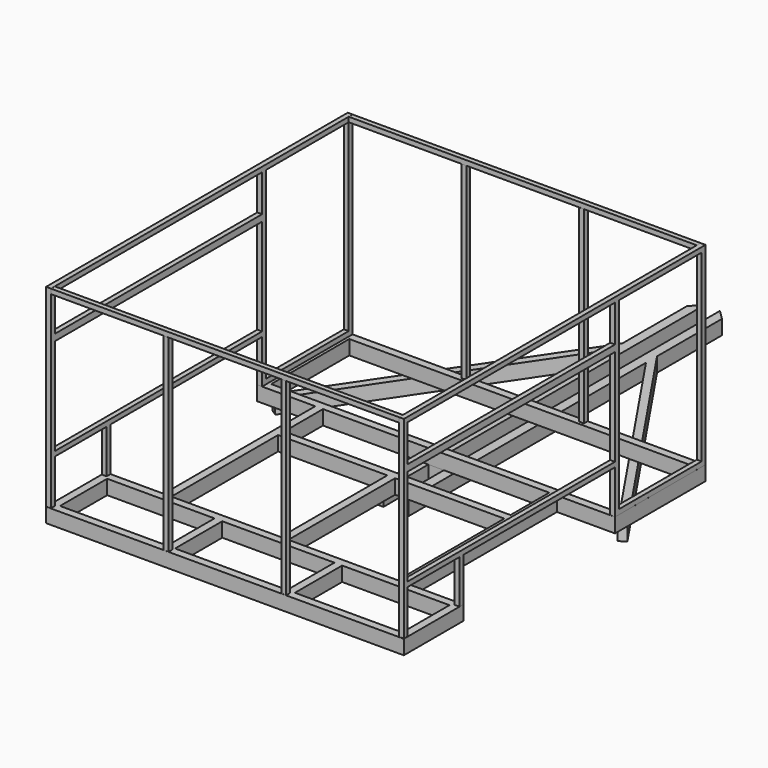
from build123d import *

# Parameters (mm, degrees)
F0_W      = 50
F0_H      = 40
F0_W_2    = 80
F0_W_3    = 495
F0_W_4    = 40
F0_H_2    = 689.5836830139
F0_H_3    = 305
F1_DEPTH  = 75
F0_H_4    = 250.4163169861
F0_H_5    = 505
F2_DEPTH  = 75
F3_W      = 535
F3_H      = 951
F3_W_2    = 25
F3_H_2    = 225.9821975827
F3_W_3    = 1340
F3_H_3    = 33.8248362541
F4_DEPTH  = 25
F7_W      = 1340
F7_H      = 33.8248362541
F7_W_2    = 535
F7_H_2    = 951
F7_W_3    = 25
F7_H_3    = 225.9821975827
F8_DEPTH  = 25
F9_W      = 25
F9_H      = 975.6403267384
F10_DEPTH = 25
F12_DEPTH = 25
F11_W     = 25
F11_H     = 975.6403267384


# Not quite as in the source:
# - a feature names something its author has since deleted; it is built from what else it names


with BuildPart() as f1:
    # F0 (on Top) → F1 (new body)
    with BuildSketch(Plane.XY):
        Polygon((341.9006320566, 0), (0, 0), (0, -585), (300, -585), (340, -585), (835, -585), (835, -545), (40, -545), (40, -518.7423229218), (6.8463404132, -496.362982985), (40, -447.2478103703), (40, -40), (314.8998843676, -40), align=None)
        Polygon((390.1607644204, 0), (341.9006320566, 0), (314.8998843676, -40), (363.1600167314, -40), align=None)
        Polygon((835, 0), (390.1607644204, 0), (363.1600167314, -40), (835, -40), align=None)
        Polygon((340, -585), (300, -585), (300, -1565), (340, -1565), (340, -875.4163169861), (340, -835.4163169861), align=None)
        with Locations((860, -20)):
            Rectangle(F0_W, F0_H)
        Polygon((40, -518.7423229218), (40, -447.2478103703), (6.8463404132, -496.362982985), align=None)
        Polygon((340, -1565), (300, -1565), (0, -1565), (0, -1950), (1850, -1950), (1850, -1565), (1550, -1565), (1510, -1565), (945, -1565), (905, -1565), align=None)
        Polygon((1255, -1605), (1810, -1605), (1810, -1910), (1255, -1910), (1215, -1910), (635, -1910), (595, -1910), (40, -1910), (40, -1605), (595, -1605), (635, -1605), (1215, -1605), align=None, mode=Mode.SUBTRACT)
        with Locations((925, -20)):
            Rectangle(F0_W_2, F0_H)
        with Locations((860, -565)):
            Rectangle(F0_W, F0_H)
        with Locations((587.5, -855.4163169861)):
            Rectangle(F0_W_3, F0_H)
        with Locations((990, -20)):
            Rectangle(F0_W, F0_H)
        with Locations((925, -565)):
            Rectangle(F0_W_2, F0_H)
        with Locations((860, -855.4163169861)):
            Rectangle(F0_W, F0_H)
        with Locations((925, -1220.208158493)):
            Rectangle(F0_W_4, F0_H_2)
        Polygon((1459.8392355796, 0), (1015, 0), (1015, -40), (1486.8399832686, -40), align=None)
        with Locations((990, -565)):
            Rectangle(F0_W, F0_H)
        Polygon((965, -835.4163169861), (885, -835.4163169861), (885, -875.4163169861), (905, -875.4163169861), (945, -875.4163169861), (965, -875.4163169861), align=None)
        Polygon((1508.0993679434, 0), (1459.8392355796, 0), (1486.8399832686, -40), (1535.1001156324, -40), align=None)
        Polygon((1015, -545), (1015, -585), (1510, -585), (1550, -585), (1850, -585), (1850, 0), (1508.0993679434, 0), (1535.1001156324, -40), (1810, -40), (1810, -447.2478103703), (1843.1536595868, -496.362982985), (1810, -518.7423229218), (1810, -545), align=None)
        with Locations((990, -855.4163169861)):
            Rectangle(F0_W, F0_H)
        Polygon((1510, -875.4163169861), (1510, -1565), (1550, -1565), (1550, -585), (1510, -585), (1510, -835.4163169861), align=None)
        with Locations((1262.5, -855.4163169861)):
            Rectangle(F0_W_3, F0_H)
        Polygon((1810, -447.2478103703), (1810, -518.7423229218), (1843.1536595868, -496.362982985), align=None)
        with Locations((1235, -1757.5)):
            Rectangle(F0_W_4, F0_H_3)
        with Locations((615, -1757.5)):
            Rectangle(F0_W_4, F0_H_3)
    extrude(amount=F1_DEPTH)


with BuildPart() as f2:
    # F0 (on Top) → F2 (new body)
    with BuildSketch(Plane.XY):
        with Locations((990, -710.208158493)):
            Rectangle(F0_W, F0_H_4)
        Polygon((835, 730.4973530704), (341.9006320566, 0), (390.1607644204, 0), (835, 659.0028405189), align=None)
        Polygon((363.1600167314, -40), (314.8998843676, -40), (40, -447.2478103703), (40, -518.7423229218), align=None)
        Polygon((390.1607644204, 0), (341.9006320566, 0), (314.8998843676, -40), (363.1600167314, -40), align=None)
        with Locations((990, -292.5)):
            Rectangle(F0_W, F0_H_5)
        Polygon((1535.1001156324, -40), (1486.8399832686, -40), (1810, -518.7423229218), (1810, -447.2478103703), align=None)
        Polygon((1015, 659.0028405189), (1459.8392355796, 0), (1508.0993679434, 0), (1015, 730.4973530704), align=None)
        Polygon((1508.0993679434, 0), (1459.8392355796, 0), (1486.8399832686, -40), (1535.1001156324, -40), align=None)
        with Locations((990, -20)):
            Rectangle(F0_W, F0_H)
        with Locations((860, -20)):
            Rectangle(F0_W, F0_H)
        with Locations((860, -565)):
            Rectangle(F0_W, F0_H)
        with Locations((925, -565)):
            Rectangle(F0_W_2, F0_H)
        with Locations((990, -565)):
            Rectangle(F0_W, F0_H)
        with Locations((860, -855.4163169861)):
            Rectangle(F0_W, F0_H)
        with Locations((990, -855.4163169861)):
            Rectangle(F0_W, F0_H)
        Polygon((40, -518.7423229218), (40, -447.2478103703), (6.8463404132, -496.362982985), align=None)
        Polygon((1810, -447.2478103703), (1810, -518.7423229218), (1843.1536595868, -496.362982985), align=None)
        with Locations((860, -292.5)):
            Rectangle(F0_W, F0_H_5)
        with Locations((860, -710.208158493)):
            Rectangle(F0_W, F0_H_4)
        Polygon((835, 1150), (835, 730.4973530704), (835, 659.0028405189), (835, 0), (885, 0), (885, 1200), align=None)
        Polygon((965, 1200), (965, 0), (1015, 0), (1015, 659.0028405189), (1015, 730.4973530704), (1015, 1150), align=None)
    extrude(amount=-F2_DEPTH)


with BuildPart() as f4:
    # F3 (on Right) → F4 (new body)
    with BuildSketch(Plane.YZ):
        Polygon((0, 75.0093311071), (0, 1076), (-1950, 1076), (-1950, 76), (-1925, 76), (-1925, 301), (-1925, 326), (-1925, 826), (-1925, 859.8248362541), (-1925, 1051), (-585, 1051), (-585, 859.8248362541), (-585, 826), (-585, 326), (-585, 301), (-585, 75.0093311071), align=None)
        with Locations((-292.5, 575.5)):
            Rectangle(F3_W, F3_H, mode=Mode.SUBTRACT)
        Polygon((-1565, 301), (-585, 301), (-585, 326), (-1925, 326), (-1925, 301), (-1590, 301), align=None)
        with Locations((-1577.5, 188.0089012086)):
            Rectangle(F3_W_2, F3_H_2)
        with Locations((-1255, 842.9124181271)):
            Rectangle(F3_W_3, F3_H_3)
    extrude(amount=F4_DEPTH)


with BuildPart() as f8:
    # F7 (on offset) → F8 (new body)
    with BuildSketch(Plane.YZ.offset(1850)):
        with Locations((-1254.9842073394, 842.9438270557)):
            Rectangle(F7_W, F7_H)
        Polygon((0.0157926606, 75.0407400358), (0.0157926606, 1076.0314089287), (-1949.9842073394, 1076.0314089287), (-1949.9842073394, 76.0314089287), (-1924.9842073394, 76.0314089287), (-1924.9842073394, 301.0314089287), (-1924.9842073394, 326.0314089287), (-1924.9842073394, 826.0314089287), (-1924.9842073394, 859.8562451828), (-1924.9842073394, 1051.0314089287), (-584.9842073394, 1051.0314089287), (-584.9842073394, 859.8562451828), (-584.9842073394, 826.0314089287), (-584.9842073394, 326.0314089287), (-584.9842073394, 301.0314089287), (-584.9842073394, 75.0407400358), align=None)
        with Locations((-292.4842073394, 575.5314089287)):
            Rectangle(F7_W_2, F7_H_2, mode=Mode.SUBTRACT)
        Polygon((-1564.9842073394, 301.0314089287), (-584.9842073394, 301.0314089287), (-584.9842073394, 326.0314089287), (-1924.9842073394, 326.0314089287), (-1924.9842073394, 301.0314089287), (-1589.9842073394, 301.0314089287), align=None)
        with Locations((-1577.4842073394, 188.0403101373)):
            Rectangle(F7_W_3, F7_H_3)
    extrude(amount=-F8_DEPTH)


with BuildPart() as f10:
    # F9 (on Front) → F10 (new body)
    with BuildSketch(Plane.XZ):
        with Locations((1229.0860442189, 563.0803654591)):
            Rectangle(F9_W, F9_H)
    extrude(amount=F10_DEPTH)


with BuildPart() as f10b:
    # F9 (on Front) → F10, piece 2 (new body)
    with BuildSketch(Plane.XZ):
        with Locations((620.7860442189, 563.0803654591)):
            Rectangle(F9_W, F9_H)
    extrude(amount=F10_DEPTH)


with BuildPart() as f10c:
    # F9 (on Front) → F10, piece 3 (new body)
    with BuildSketch(Plane.XZ):
        Polygon((25.0013015178, 1075.9552220504), (24.9906565008, 1050.9557227294), (1824.9834692982, 1050.9557227294), (1824.9834692982, 1076.006124417), align=None)
    extrude(amount=F10_DEPTH)


with BuildPart() as f12:
    # F11 (on offset) → F12 (new body)
    with BuildSketch(Plane.XZ.offset(1950)):
        Polygon((25.0165007023, 1075.9785572688), (25.0058556852, 1050.9790579478), (1824.9986684827, 1050.9790579478), (1824.9986684827, 1076.0294596354), align=None)
    extrude(amount=-F12_DEPTH)


with BuildPart() as f12b:
    # F11 (on offset) → F12, piece 2 (new body)
    with BuildSketch(Plane.XZ.offset(1950)):
        with Locations((620.8012434033, 563.1037006776)):
            Rectangle(F11_W, F11_H)
    extrude(amount=-F12_DEPTH)


with BuildPart() as f12c:
    # F11 (on offset) → F12, piece 3 (new body)
    with BuildSketch(Plane.XZ.offset(1950)):
        with Locations((1229.1012434033, 563.1037006776)):
            Rectangle(F11_W, F11_H)
    extrude(amount=-F12_DEPTH)


solid = Compound([f1.part, f2.part, f4.part, f8.part, f10.part, f10b.part, f10c.part, f12.part, f12b.part, f12c.part])
